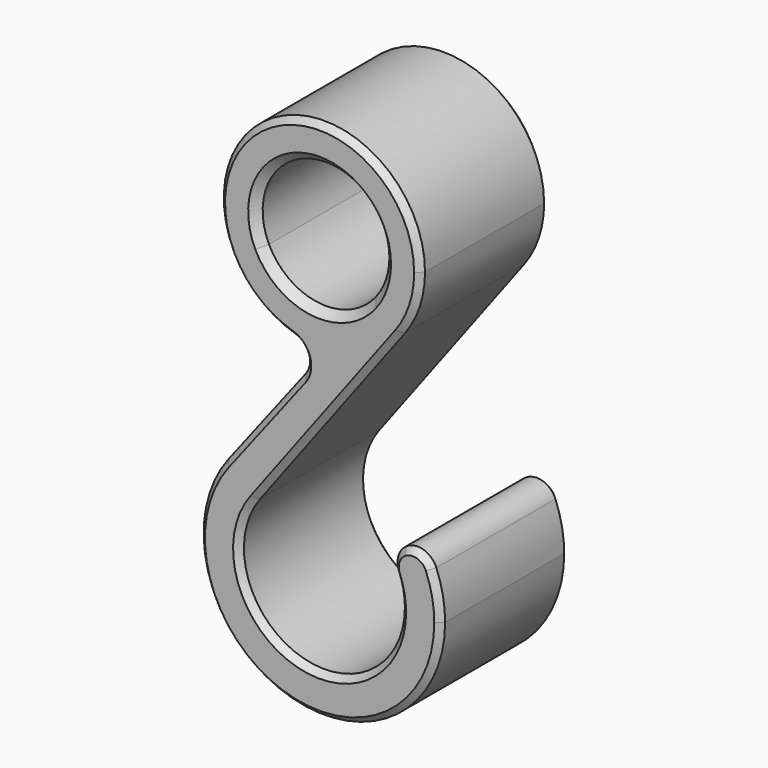
from build123d import *

# Parameters (mm, degrees)
F1_DEPTH = 16
F2_R     = 1.99999
F3_SIZE  = 0.8
F4_SIZE  = 0.6


# Not quite as in the source:
# - a fillet or chamfer is up to 0.001 mm smaller than in the source, because OpenCascade refuses the exact size


with BuildPart() as f1:
    # F0 (on Front) → F1 (new body)
    with BuildSketch(Plane.XZ):
        with BuildLine():
            ThreePointArc((6.3, 0), (5.9640762947, -2.0297275557), (4.9921289046, -3.843))
            Line((4.9921289046, -3.843), (0.2548985956, -9.9967508074))
            ThreePointArc((0.2548985956, -9.9967508074), (4.5857760478, -8.8865436498), (8, -6))
            ThreePointArc((8, -6), (9.4868329805, -3.1622776602), (10, 0))
            ThreePointArc((10, 0), (-2.2360679775, 9.7467943448), (-9, -4.3588989435))
            Line((-9, -4.3588989435), (-5.67, -2.7461063344))
            ThreePointArc((-5.67, -2.7461063344), (-1.4087228258, 6.1404804372), (6.3, 0))
        make_face()
        with BuildLine():
            ThreePointArc((8, -6), (4.5857760478, -8.8865436498), (0.2548985956, -9.9967508074))
            Line((0.2548985956, -9.9967508074), (-9.5088169611, -22.68))
            ThreePointArc((-9.5088169611, -22.68), (-5.7581726954, -19.4717785353), (-1.033436854, -18.044582472))
            Line((-1.033436854, -18.044582472), (8, -6))
        make_face()
        with BuildLine():
            ThreePointArc((-1.033436854, -18.044582472), (-5.7581726954, -19.4717785353), (-9.5088169611, -22.68))
            ThreePointArc((-9.5088169611, -22.68), (-3.8661477252, -41.3601453233), (12, -30))
            ThreePointArc((12, -30), (11.4891252931, -26.5358983849), (10, -23.3667504193))
            Line((10, -23.3667504193), (6.6666666667, -25.5778336129))
            ThreePointArc((6.6666666667, -25.5778336129), (7.6594168621, -27.6905989232), (8, -30))
            ThreePointArc((8, -30), (-2.5298221281, -37.5894663844), (-6.4, -25.2))
            Line((-6.4, -25.2), (-1.033436854, -18.044582472))
        make_face()
        with BuildLine():
            Line((0.2548985956, -9.9967508074), (4.9921289046, -3.843))
            ThreePointArc((4.9921289046, -3.843), (-0.6447257044, -6.2669233892), (-5.67, -2.7461063344))
            Line((-5.67, -2.7461063344), (-9, -4.3588989435))
            ThreePointArc((-9, -4.3588989435), (-5.202455483, -8.5401672669), (0.2548985956, -9.9967508074))
        make_face()
    extrude(amount=F1_DEPTH)

    # F2 (radius 2 in the source; OpenCascade refuses exactly that, so slightly less here)
    f2_edges = [f1.edges().sort_by_distance(p)[0] for p in [
        (4.992129, -8, -3.843),
        (8, -8, -6),
        (10, -8, -23.36675),
        (6.666667, -8, -25.577834),
        (0.254899, -8, -9.996751),
    ]]
    fillet(f2_edges, radius=F2_R)

    # F3
    f3_edges = [f1.edges().sort_by_distance(p)[0] for p in [
        (-4.992129, -16, 3.843),
        (-4.992129, 0, 3.843),
    ]]
    chamfer(f3_edges, length=F3_SIZE)

    # F4
    f4_edges = [f1.edges().sort_by_distance(p)[0] for p in [
        (-3.134832, -16, 9.495937),
        (0.8, 0, -15.6),
        (-5.675293, 0, -17.70018),
        (-1.523485, 0, -10.885342),
        (-1.625379, 0, -41.889413),
        (-3.134832, 0, 9.495937),
        (9.862297, 0, -24.340194),
        (8.164968, 0, -24.583973),
        (-1.033792, 0, -37.932923),
        (7.360063, 0, -25.658852),
        (-5.675293, -16, -17.70018),
        (-1.523485, -16, -10.885342),
        (-1.625379, -16, -41.889413),
        (9.862297, -16, -24.340194),
        (0.8, -16, -15.6),
        (8.164968, -16, -24.583973),
        (-1.033792, -16, -37.932923),
        (7.360063, -16, -25.658852),
    ]]
    chamfer(f4_edges, length=F4_SIZE)


solid = f1.part
